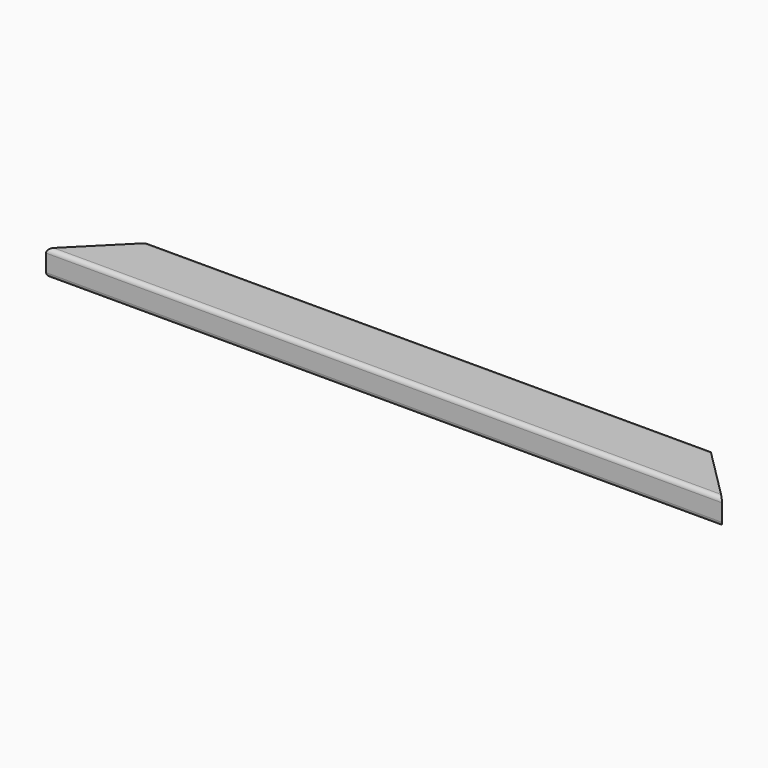
from build123d import *

# Parameters (mm, degrees)
F1_DEPTH = 558.8
F3_DEPTH = 19.178
F5_DEPTH = 19.178
F7_DEPTH = 19.178


with BuildPart() as f1:
    # F0 (on Right) → F1 (new body)
    with BuildSketch(Plane.YZ):
        with BuildLine():
            Line((-11.0857636662, 35.1864280597), (-48.1697636662, 35.1864280597))
            ThreePointArc((-48.1697636662, 35.1864280597), (-50.4148276965, 34.25649209), (-51.3447636662, 32.0114280597))
            Line((-51.3447636662, 32.0114280597), (-51.3447636662, 19.1844280597))
            ThreePointArc((-51.3447636662, 19.1844280597), (-50.4148276965, 16.9393640294), (-48.1697636662, 16.0094280597))
            Line((-48.1697636662, 16.0094280597), (-15.9117636662, 16.0094280597))
            Line((-15.9117636662, 16.0094280597), (-15.9117636662, 24.8994280597))
            Line((-15.9117636662, 24.8994280597), (-7.9107636662, 24.8994280597))
            Line((-7.9107636662, 24.8994280597), (-7.9107636662, 32.0114280597))
            ThreePointArc((-7.9107636662, 32.0114280597), (-8.8406996359, 34.25649209), (-11.0857636662, 35.1864280597))
        make_face()
    extrude(amount=F1_DEPTH)

    # F2 (on face) → F3 (cut, through all)
    with BuildSketch(Plane.XY.offset(35.1864280597)):
        Polygon((0, -11.0857636662), (40.259, -11.0857636662), (43.434, -7.9107636662), (0, -7.9107636662), align=None)
        Polygon((0, -48.1697636662), (3.175, -48.1697636662), (40.259, -11.0857636662), (0, -11.0857636662), align=None)
        Polygon((0, -48.1697636662), (0, -51.3447636662), (3.175, -48.1697636662), align=None)
    extrude(amount=-F3_DEPTH, mode=Mode.SUBTRACT)

    # F4 (on face) → F5 (cut, through all)
    with BuildSketch(Plane(origin=(0, 0, 16.0094280597), x_dir=(1, 0, 0), z_dir=(0, 0, -1))):
        Polygon((558.8, 48.1697636662), (558.8, 51.3447636662), (521.843, 51.3447636662), (518.668, 48.1697636662), align=None)
        Polygon((558.8, 15.9117636662), (558.8, 48.1697636662), (518.668, 48.1697636662), (486.41, 15.9117636662), align=None)
        Polygon((558.8, 7.9107636662), (558.8, 15.9117636662), (486.41, 15.9117636662), (478.409, 7.9107636662), align=None)
    extrude(amount=-F5_DEPTH, mode=Mode.SUBTRACT)

    # F6 (on face) → F7 (cut, through all)
    with BuildSketch(Plane(origin=(0, 0, 16.0094280597), x_dir=(1, 0, 0), z_dir=(0, 0, -1))):
        Polygon((470.408, 15.9117636662), (470.408, 15.5282095075), (470.408, 14.7099299356), (470.408, 7.9107636662), (478.409, 7.9107636662), (486.41, 15.9117636662), align=None)
        Polygon((470.408, 14.7099299356), (470.408, 15.5282095075), (470.408, 15.9117636662), (462.407, 7.9107636662), (470.408, 7.9107636662), align=None)
        Polygon((502.666, 48.1697636662), (470.408, 15.9117636662), (486.41, 15.9117636662), (518.668, 48.1697636662), align=None)
        Polygon((505.841, 51.3447636662), (502.666, 48.1697636662), (518.668, 48.1697636662), (521.843, 51.3447636662), align=None)
    extrude(amount=-F7_DEPTH, mode=Mode.SUBTRACT)


solid = f1.part
